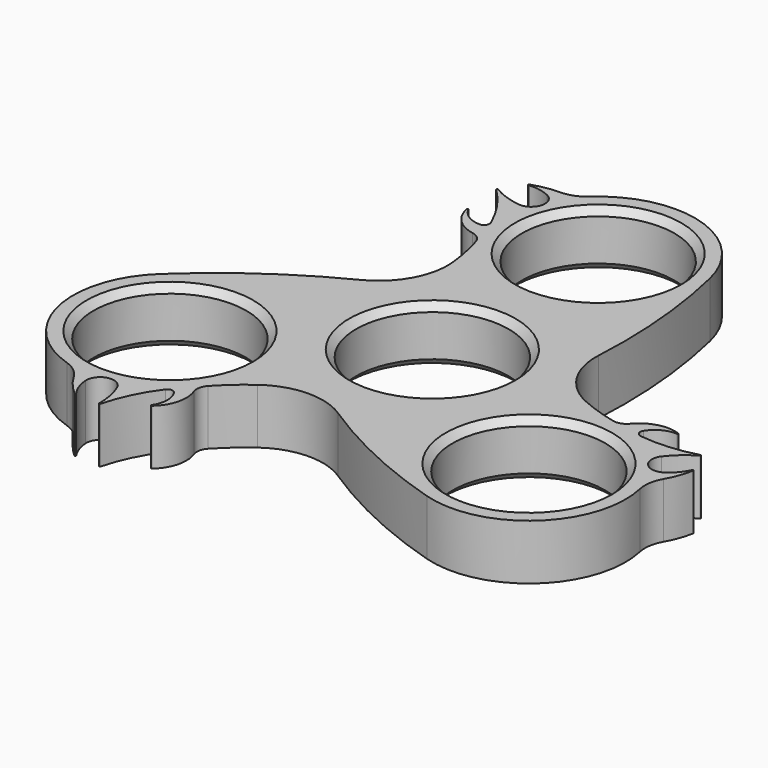
from build123d import *

# Parameters (mm, degrees)
F0_R     = 11.05
F1_DEPTH = 8
F2_COUNT = 3
F3_R     = 10
F4_R     = 5
F5_SIZE  = 1


with BuildPart() as f1:
    # F0 (on Top) → F1 (new body)
    with BuildSketch(Plane.XY):
        with BuildLine():
            ThreePointArc((-12.6514260567, 23.6933629251), (-11.3751248169, 14.1917767316), (-13.1613477418, 4.7727272727))
            ThreePointArc((-13.1613477418, 4.7727272727), (-3.9842769003, -13.421085559), (13.6336360909, -3.1818181818))
            ThreePointArc((13.6336360909, -3.1818181818), (15.7271441431, 15), (13.6336360909, 33.1818181818))
            ThreePointArc((13.6336360909, 33.1818181818), (3.1856807408, 43.6327340698), (-10.8117310602, 38.8941818894))
            ThreePointArc((-10.8117310602, 38.8941818894), (-13.7694685953, 39.0065439815), (-16.6610679634, 38.374492037))
            ThreePointArc((-16.6610679634, 38.374492037), (-16.7251928987, 38.2586862032), (-16.6182205389, 38.1807124082))
            ThreePointArc((-16.6182205389, 38.1807124082), (-14.990242489, 38.1077523786), (-13.4439973475, 37.5932024207))
            ThreePointArc((-13.4439973475, 37.5932024207), (-12.4179647139, 35.2171421288), (-14.5954308534, 33.8181972809))
            ThreePointArc((-14.5954308534, 33.8181972809), (-16.7144110874, 34.3205676404), (-18.6910590274, 35.2345239477))
            ThreePointArc((-18.6910590274, 35.2345239477), (-18.82124029, 35.2092689611), (-18.8118896462, 35.0769906902))
            ThreePointArc((-18.8118896462, 35.0769906902), (-16.1822484317, 31.9388495716), (-14.2139807274, 28.3487430493))
            ThreePointArc((-14.2139807274, 28.3487430493), (-14.2850540536, 27.5953224844), (-14.9557406683, 27.2447894188))
            ThreePointArc((-14.9557406683, 27.2447894188), (-16.8849368279, 27.8185608598), (-18.2353559933, 29.311001668))
            ThreePointArc((-18.2353559933, 29.311001668), (-18.3566059607, 29.361220693), (-18.4231712091, 29.2481164368))
            ThreePointArc((-18.4231712091, 29.2481164368), (-16.9723331855, 26.5082159897), (-14.218759745, 25.0834989167))
            ThreePointArc((-14.218759745, 25.0834989167), (-13.2385127521, 24.6100687257), (-12.6514260567, 23.6933629251))
        make_face()
        Circle(F0_R, mode=Mode.SUBTRACT)
        with Locations((0, 30)):
            Circle(F0_R, mode=Mode.SUBTRACT)
    extrude(amount=F1_DEPTH)

    # F2: F1 ×3 about axis
    f2_axis = Axis((0, 0, 0), (0, 0, -1))


with BuildPart() as f1_1:
    add(f1.part)
    for i in range(1, F2_COUNT):
        add(f1.part.rotate(f2_axis, i * 360 / F2_COUNT))

    # F3
    f3_edges = [f1_1.edges().sort_by_distance(p)[0] for p in [
        (15.072251, 4.78462, 4),
        (-3.392523, -15.445263, 4),
        (-11.679728, 10.660642, 4),
    ]]
    fillet(f3_edges, radius=F3_R)

    # F4
    f4_edges = [f1_1.edges().sort_by_distance(p)[0] for p in [
        (-28.277484, -28.810325, 4),
        (39.089215, -10.083857, 4),
        (-10.811731, 38.894182, 4),
    ]]
    fillet(f4_edges, radius=F4_R)

    # F5
    f5_edges = [f1_1.edges().sort_by_distance(p)[0] for p in [
        (-11.05, 30, 8),
        (-11.05, 30, 0),
        (-11.05, 0, 8),
        (-11.05, 0, 0),
        (31.505762, -5.430419, 8),
        (31.505762, -5.430419, 0),
        (-20.455762, -24.569581, 8),
        (-20.455762, -24.569581, 0),
    ]]
    chamfer(f5_edges, length=F5_SIZE)


solid = f1_1.part
